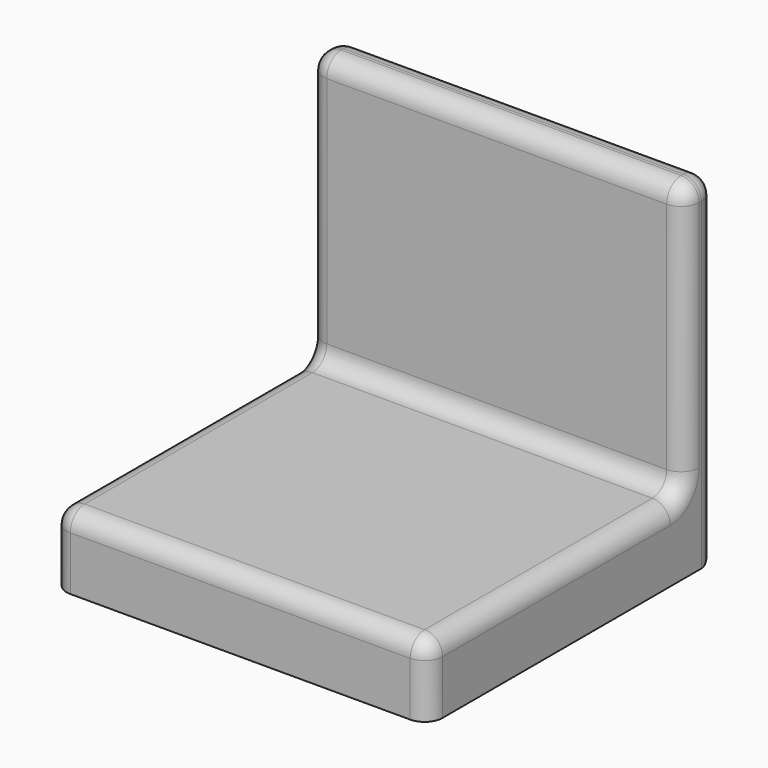
from build123d import *

# Parameters (mm, degrees)
F0_W     = 209.176
F0_H     = 200
F1_DEPTH = 40
F2_W     = 209.176
F2_H     = 21.5614646673
F3_DEPTH = 150
F4_R     = 10
F5_DEPTH = 20
F6_F1_R  = 10
F6_F2_R  = 10
F7_R     = 10


with BuildPart() as f1:
    # F0 (on Top) → F1 (new body)
    with BuildSketch(Plane.XY):
        Rectangle(F0_W, F0_H)
    extrude(amount=F1_DEPTH)

    # F2 (on face) → F3 (join)
    with BuildSketch(Plane.XY.offset(40)):
        with Locations((0, 89.2192676663)):
            Rectangle(F2_W, F2_H)
    extrude(amount=F3_DEPTH)

    # F4 (on face) → F5 (cut)
    with BuildSketch(Plane(origin=(0, 0, 0), x_dir=(1, 0, 0), z_dir=(0, 0, -1))):
        Circle(F4_R)
    extrude(amount=-F5_DEPTH, mode=Mode.SUBTRACT)

    # F6: fillet of radius 10 on 10 edges, made by hand

    # F6_f1
    f6_f1_edges = [f1.edges().sort_by_distance(p)[0] for p in [
        (0, 78.4385353327, 40),
    ]]
    fillet(f6_f1_edges, radius=F6_F1_R)

    # F6_f2
    f6_f2_edges = [f1.edges().sort_by_distance(p)[0] for p in [
        (0, 78.4385353327, 190),
        (0, 100, 190),
        (-104.588, 89.2192676663, 190),
        (104.588, 89.2192676663, 190),
        (-104.588, 78.4385353327, 120),
        (104.588, 78.4385353327, 120),
        (104.588, 100, 95),
        (-104.588, 100, 95),
        (0, 100, 0),
        (104.588, 75.5096031445, 42.9289321881),
        (-104.588, 75.5096031445, 42.9289321881),
    ]]
    fillet(f6_f2_edges, radius=F6_F2_R)

    # F7
    f7_edges = [f1.edges().sort_by_distance(p)[0] for p in [
        (0, -100, 40),
    ]]
    fillet(f7_edges, radius=F7_R)


solid = f1.part
